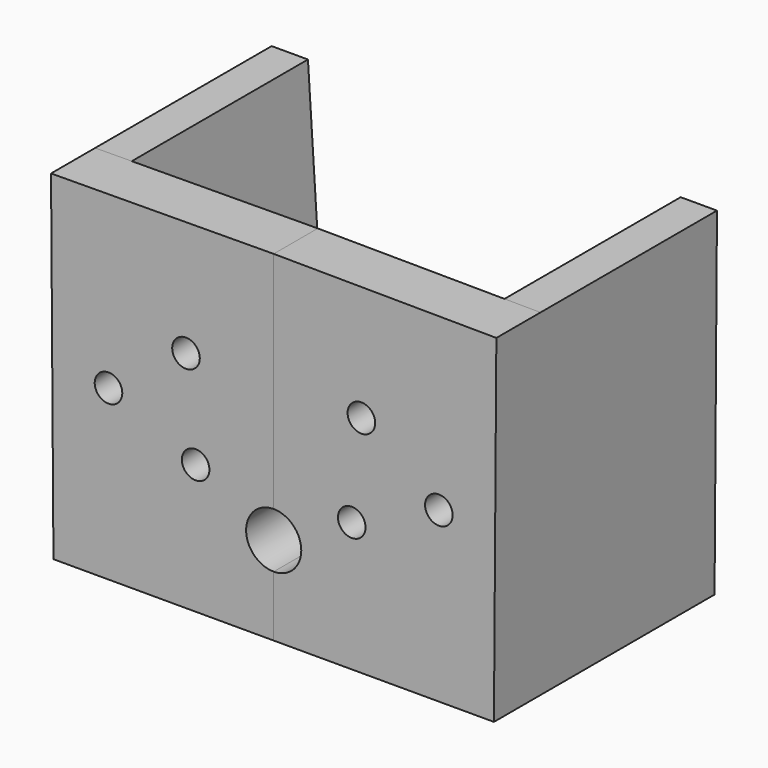
from build123d import *
from build123d import SkipClean  # not in build123d's __all__

# Parameters (mm, degrees)
F1_DEPTH = 20
F3_DEPTH = 5
F4_D     = 2.5
F4_DEPTH = 5.001


with BuildPart() as f1:
    # F0 (on Front) → F1 (new body)
    with BuildSketch(Plane.XZ):
        Polygon((-19.9654586613, 0), (0, 0), (0, 3.0716089532), (-15.1386437938, 3.0716089532), (-16.8938487768, 30.7160895318), (-20.1848596334, 30.7160895318), align=None)
    extrude(amount=F1_DEPTH)

    # F2 (on face) → F3 (join)
    with BuildSketch(Plane.XZ.offset(20)):
        with BuildLine():
            Line((0, 30.8602673192), (-20.1848596334, 30.7160895318))
            Line((-20.1848596334, 30.7160895318), (-16.8938487768, 30.7160895318))
            Line((-16.8938487768, 30.7160895318), (-15.1386437938, 3.0716089532))
            Line((-15.1386437938, 3.0716089532), (0, 3.0716089532))
            Line((0, 3.0716089532), (0, 5.4992720857))
            ThreePointArc((0, 5.4992720857), (-2.5, 7.9992720857), (0, 10.4992720857))
            Line((0, 10.4992720857), (0, 30.8602673192))
        make_face()
        Polygon((-16.8938487768, 30.7160895318), (-20.1848596334, 30.7160895318), (-19.9654586613, 0), (0, 0), (0, 3.0716089532), (-15.1386437938, 3.0716089532), align=None)
    extrude(amount=F3_DEPTH)

    # F4 (through all, one way)
    with BuildSketch(Plane(origin=(0, -20, 0), x_dir=(1, 0, 0), z_dir=(0, 1, 0))):
        with Locations((-14.9744828703, -15.2839560666), (-7.0758488149, -11.7326774155), (-7.9496683148, -20.3487344883)):
            Circle(F4_D / 2)
    extrude(amount=-F4_DEPTH, mode=Mode.SUBTRACT)

    # F5: F1 across plane


with BuildPart() as f1_1:
    add(f1.part, clean=False)
    with SkipClean():  # cleaning this boolean's faces spoils the solid; the shape is the same uncleaned
        add(f1.part.mirror(Plane.YZ), clean=False)


solid = f1_1.part
